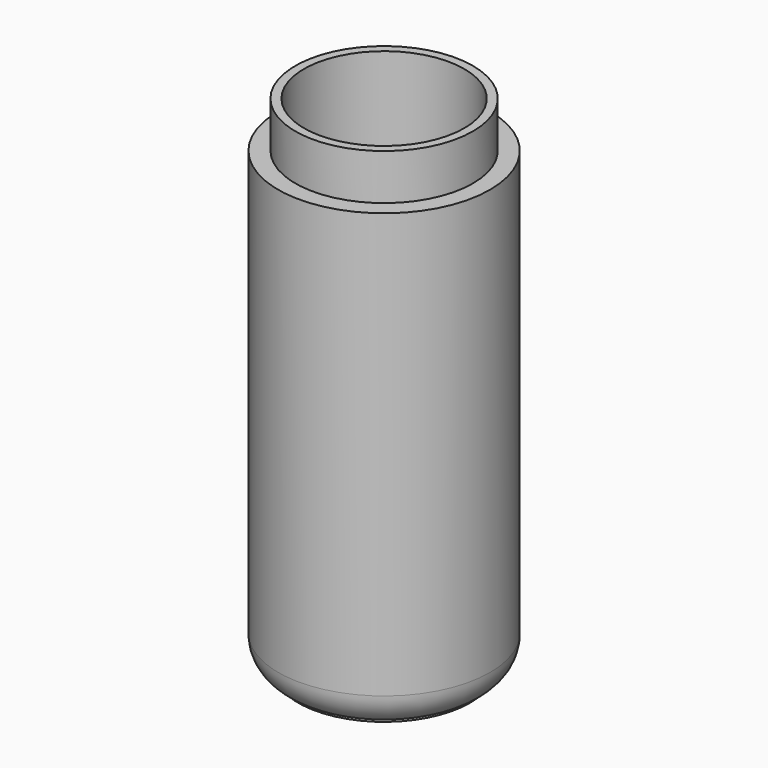
from build123d import *

# Parameters (mm, degrees)
F0_R     = 9.25
F0_R_2   = 7
F1_DEPTH = 40
F2_R     = 7.5
F4_DEPTH = 2
F5_R     = 7.75
F5_R_2   = 7
F6_DEPTH = 4


# Not quite as in the source:
# - a fillet or chamfer that OpenCascade refuses, or shapes differently, is made with other operations: its cross-section is extruded or revolved along the edge and cut away or added


with BuildPart() as f1:
    # F0 (on Top) → F1 (new body)
    with BuildSketch(Plane.XY):
        Circle(F0_R)
        Circle(F0_R_2, mode=Mode.SUBTRACT)
    extrude(amount=F1_DEPTH)

    # F3: fillet of radius 3 on 1 edges, made by hand

    # F3_s1 → F3_t2 (revolve, cut)
    with BuildSketch(Plane.XZ):
        with BuildLine():
            ThreePointArc((9.25, 2.9047375097), (8.6217082451, 1.0676202026), (7, 0))
            Line((7, 0), (9.25, 0))
            Line((9.25, 0), (9.25, 2.9047375097))
        make_face()
    revolve(axis=Axis((0, 0, 0), (0, 0, 1)), mode=Mode.SUBTRACT)

    # F2 (on face) → F4 (join)
    with BuildSketch(Plane(origin=(0, 0, 0), x_dir=(1, 0, 0), z_dir=(0, 0, -1))):
        Circle(F2_R)
    extrude(amount=-F4_DEPTH)

    # F5 (on face) → F6 (join)
    with BuildSketch(Plane.XY.offset(40)):
        Circle(F5_R)
        Circle(F5_R_2, mode=Mode.SUBTRACT)
    extrude(amount=F6_DEPTH)


solid = f1.part
